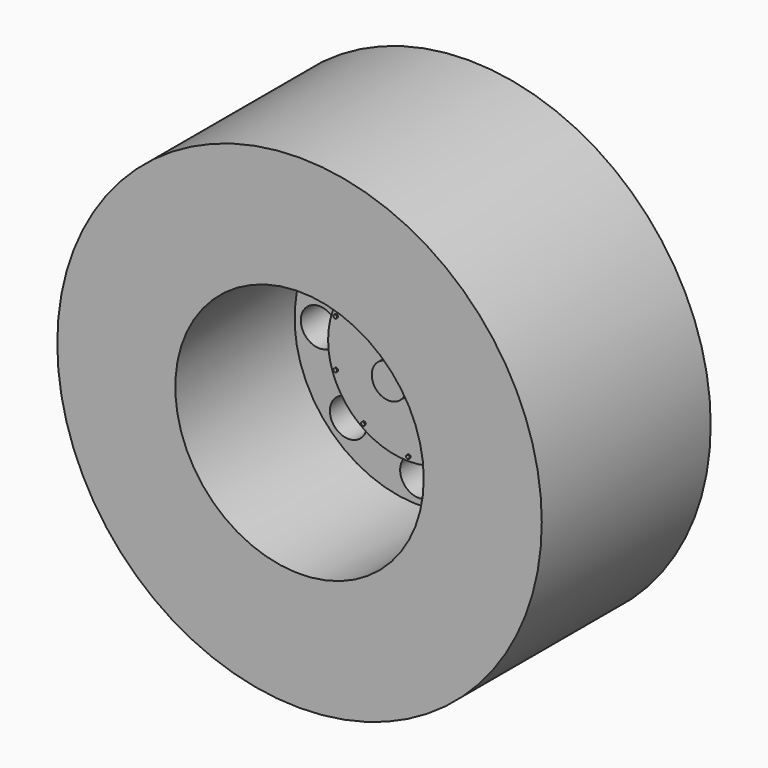
from build123d import *

# Parameters (mm, degrees)
F0_R      = 19.5
F1_DEPTH  = 17
F2_R      = 10
F3_DEPTH  = 12
F4_R      = 1.5
F5_DEPTH  = 25
F6_R      = 6.5
F7_DEPTH  = 1
F8_R      = 0.1455076687
F9_DEPTH  = 0.1
F11_R     = 1.3872068032
F12_DEPTH = 2
F13_R     = 2.3581013166
F14_DEPTH = 7
F15_R     = 0.8149743097
F16_DEPTH = 13.4


with BuildPart() as f1:
    # F0 (on Front) → F1 (new body)
    with BuildSketch(Plane.XZ):
        Circle(F0_R)
    extrude(amount=F1_DEPTH)

    # F2 (on face) → F3 (cut)
    with BuildSketch(Plane.XZ.offset(17)):
        Circle(F2_R)
    extrude(amount=-F3_DEPTH, mode=Mode.SUBTRACT)

    # F4 (on face) → F5 (cut)
    with BuildSketch(Plane(origin=(0, 0, 0), x_dir=(-1, 0, 0), z_dir=(0, 1, 0))):
        with BuildLine():
            ThreePointArc((0, 9.5), (-1.5, 8), (0, 6.5))
            ThreePointArc((0, 6.5), (1.0606601718, 6.9393398282), (1.5, 8))
            ThreePointArc((1.5, 8), (1.0606601718, 9.0606601718), (0, 9.5))
        make_face()
        with Locations((-5.6568542495, 5.6568542495)):
            Circle(F4_R)
        with Locations((-8, 0)):
            Circle(F4_R)
        with Locations((-5.6568542495, -5.6568542495)):
            Circle(F4_R)
        with Locations((0, -8)):
            Circle(F4_R)
        with Locations((5.6568542495, -5.6568542495)):
            Circle(F4_R)
        with Locations((8, 0)):
            Circle(F4_R)
        with Locations((5.6568542495, 5.6568542495)):
            Circle(F4_R)
    extrude(amount=-F5_DEPTH, mode=Mode.SUBTRACT)

    # F6 (on face) → F7 (join)
    with BuildSketch(Plane.XZ.offset(5)):
        Circle(F6_R)
        with BuildLine():
            ThreePointArc((4.5961940604, -4.596194095), (6.0052169566, -2.4874423217), (6.5, 0))
            ThreePointArc((6.5, 0), (6.0052169613, 2.4874423104), (4.5961940777, 4.5961940777))
            ThreePointArc((4.5961940777, 4.5961940777), (2.4874423104, 6.0052169613), (0, 6.5))
            ThreePointArc((0, 6.5), (-2.4874423043, 6.0052169639), (-4.5961940684, 4.5961940871))
            ThreePointArc((-4.5961940684, 4.5961940871), (-6.0052169588, 2.4874423165), (-6.5, 0))
            ThreePointArc((-6.5, 0), (-6.0052169618, -2.4874423093), (-4.5961940793, -4.5961940761))
            ThreePointArc((-4.5961940793, -4.5961940761), (-2.4874423124, -6.0052169605), (-2.2e-09, -6.5))
            ThreePointArc((-2.2e-09, -6.5), (2.487442298, -6.0052169664), (4.5961940604, -4.596194095))
        make_face()
    extrude(amount=F7_DEPTH)

    # F8 (on face) → F9 (join)
    with BuildSketch(Plane.XZ.offset(6)):
        with Locations((0, 6.145354826)):
            Circle(F8_R)
        with Locations((-3.6121489368, 4.9716964907)):
            Circle(F8_R)
        with Locations((-5.8445797522, 1.8990190777)):
            Circle(F8_R)
        with Locations((-5.8445797522, -1.8990190777)):
            Circle(F8_R)
        with Locations((-3.6121489368, -4.9716964907)):
            Circle(F8_R)
        with Locations((0, -6.145354826)):
            Circle(F8_R)
        with Locations((3.6121489368, -4.9716964907)):
            Circle(F8_R)
        with Locations((5.8445797522, -1.8990190777)):
            Circle(F8_R)
        with Locations((5.8445797522, 1.8990190777)):
            Circle(F8_R)
        with Locations((3.6121489368, 4.9716964907)):
            Circle(F8_R)
    extrude(amount=F9_DEPTH)

    # F11 (on face) → F12 (join)
    with BuildSketch(Plane.XZ.offset(6)):
        Circle(F11_R)
    extrude(amount=F12_DEPTH)

    # F13 (on face) → F14 (join)
    with BuildSketch(Plane(origin=(0, 0, 0), x_dir=(-1, 0, 0), z_dir=(0, 1, 0))):
        Circle(F13_R)
    extrude(amount=F14_DEPTH)

    # F15 (on face) → F16 (cut)
    with BuildSketch(Plane(origin=(0, 7, 0), x_dir=(-1, 0, 0), z_dir=(0, 1, 0))):
        Circle(F15_R)
    extrude(amount=-F16_DEPTH, mode=Mode.SUBTRACT)


solid = f1.part
